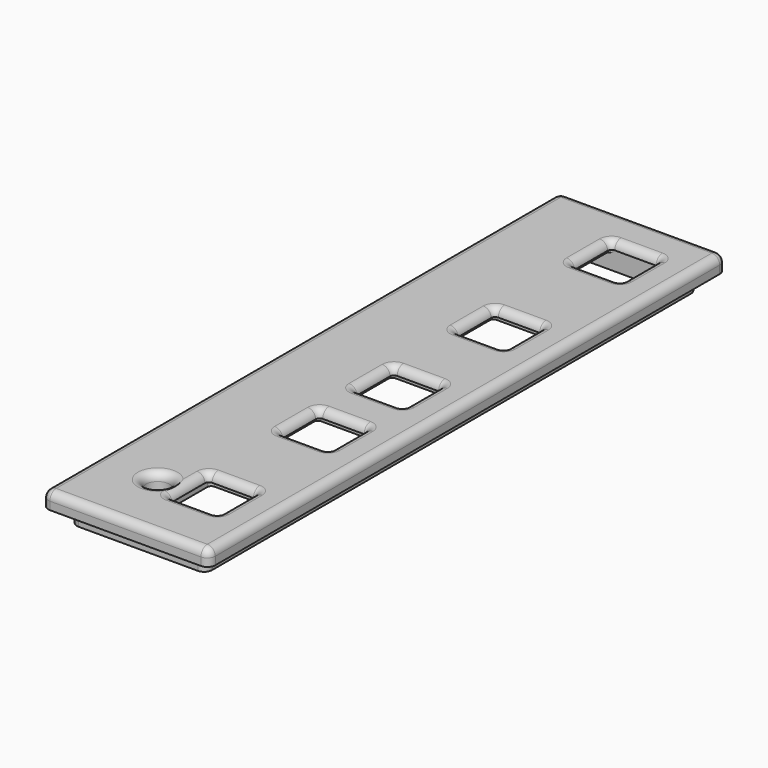
from build123d import *

# Parameters (mm, degrees)
F0_W          = 21
F0_H          = 81.3
F0_W_2        = 17
F0_H_2        = 77.3
F0_W_3        = 13
F0_H_3        = 73.3
F1_DEPTH      = 2
F2_DEPTH      = 2
F3_R          = 1.5
F4_DEPTH      = 25
F5_T1_DEPTH   = 79.3
F5_T3_DEPTH   = 19
F5_T5_DEPTH   = 5.2
F5_T7_DEPTH   = 5.2
F5_T9_DEPTH   = 5.2
F5_T11_DEPTH  = 5.2
F5_T13_DEPTH  = 5.2
F5_T15_DEPTH  = 5.2
F5_T17_DEPTH  = 3.5
F5_T19_DEPTH  = 4.5
F5_S23_W      = 1
F5_S23_H      = 1
F5_T24_DEPTH  = 1
F5_S29_W      = 1
F5_S29_H      = 1
F5_T30_DEPTH  = 1
F5_S35_W      = 1
F5_S35_H      = 1
F5_T36_DEPTH  = 1
F5_S41_W      = 1
F5_S41_H      = 1
F5_T42_DEPTH  = 1
F5_T48_ANGLE  = 90
F5_T50_ANGLE  = 90
F5_T52_ANGLE  = 90
F5_T54_ANGLE  = 90
F5_T56_ANGLE  = 90
F5_T58_ANGLE  = 90
F5_T60_ANGLE  = 90
F5_T62_ANGLE  = 90
F5_T64_ANGLE  = 90
F5_T66_ANGLE  = 90
F5_T68_ANGLE  = 90
F5_T70_ANGLE  = 90
F5_T72_ANGLE  = 90
F5_T74_ANGLE  = 90
F5_T76_ANGLE  = 90
F5_T78_ANGLE  = 90
F5_T80_ANGLE  = 90
F5_T82_ANGLE  = 90
F5_T84_ANGLE  = 90
F5_T86_ANGLE  = 90
F7_DEPTH      = 1
F7_DEPTH_BACK = 3


# Not quite as in the source:
# - a fillet or chamfer that OpenCascade refuses, or shapes differently, is made with other operations: its cross-section is extruded or revolved along the edge and cut away or added


with BuildPart() as f1:
    # F0 (on Top) → F1 (new body)
    with BuildSketch(Plane.XY):
        Rectangle(F0_W, F0_H)
        Rectangle(F0_W_2, F0_H_2, mode=Mode.SUBTRACT)
        Rectangle(F0_W_2, F0_H_2)
        Rectangle(F0_W_3, F0_H_3, mode=Mode.SUBTRACT)
        Rectangle(F0_W_3, F0_H_3)
    extrude(amount=F1_DEPTH)

    # F0 (on Top) → F2 (join)
    with BuildSketch(Plane.XY):
        Rectangle(F0_W_2, F0_H_2)
        Rectangle(F0_W_3, F0_H_3, mode=Mode.SUBTRACT)
    extrude(amount=-F2_DEPTH)

    # F3 (on face) → F4 (cut)
    with BuildSketch(Plane.XY.offset(2)):
        with BuildLine():
            ThreePointArc((6.2, 35.15), (6.0535533906, 35.5035533906), (5.7, 35.65))
            Line((5.7, 35.65), (0.5, 35.65))
            ThreePointArc((0.5, 35.65), (0.1464466094, 35.5035533906), (0, 35.15))
            Line((0, 35.15), (0, 29.95))
            ThreePointArc((0, 29.95), (0.1464466094, 29.5964466094), (0.5, 29.45))
            Line((0.5, 29.45), (5.7, 29.45))
            ThreePointArc((5.7, 29.45), (6.0535533906, 29.5964466094), (6.2, 29.95))
            Line((6.2, 29.95), (6.2, 35.15))
        make_face()
        with BuildLine():
            ThreePointArc((6.2, 16.85), (6.0535533906, 17.2035533906), (5.7, 17.35))
            Line((5.7, 17.35), (0.5, 17.35))
            ThreePointArc((0.5, 17.35), (0.1464466094, 17.2035533906), (0, 16.85))
            Line((0, 16.85), (0, 11.65))
            ThreePointArc((0, 11.65), (0.1464466094, 11.2964466094), (0.5, 11.15))
            Line((0.5, 11.15), (5.7, 11.15))
            ThreePointArc((5.7, 11.15), (6.0535533906, 11.2964466094), (6.2, 11.65))
            Line((6.2, 11.65), (6.2, 16.85))
        make_face()
        with BuildLine():
            Line((5.7, 1.45), (0.5, 1.45))
            ThreePointArc((0.5, 1.45), (0.1464466094, 1.3035533906), (0, 0.95))
            Line((0, 0.95), (0, -4.25))
            ThreePointArc((0, -4.25), (0.1464466094, -4.6035533906), (0.5, -4.75))
            Line((0.5, -4.75), (5.7, -4.75))
            ThreePointArc((5.7, -4.75), (6.0535533906, -4.6035533906), (6.2, -4.25))
            Line((6.2, -4.25), (6.2, 0.95))
            ThreePointArc((6.2, 0.95), (6.0535533906, 1.3035533906), (5.7, 1.45))
        make_face()
        with BuildLine():
            ThreePointArc((6.2, -10.75), (6.0535533906, -10.3964466094), (5.7, -10.25))
            Line((5.7, -10.25), (0.5, -10.25))
            ThreePointArc((0.5, -10.25), (0.1464466094, -10.3964466094), (0, -10.75))
            Line((0, -10.75), (0, -15.95))
            ThreePointArc((0, -15.95), (0.1464466094, -16.3035533906), (0.5, -16.45))
            Line((0.5, -16.45), (5.7, -16.45))
            ThreePointArc((5.7, -16.45), (6.0535533906, -16.3035533906), (6.2, -15.95))
            Line((6.2, -15.95), (6.2, -10.75))
        make_face()
        with BuildLine():
            ThreePointArc((6.2, -28.15), (6.0535533906, -27.7964466094), (5.7, -27.65))
            Line((5.7, -27.65), (0.5, -27.65))
            ThreePointArc((0.5, -27.65), (0.1464466094, -27.7964466094), (0, -28.15))
            Line((0, -28.15), (0, -33.35))
            ThreePointArc((0, -33.35), (0.1464466094, -33.7035533906), (0.5, -33.85))
            Line((0.5, -33.85), (5.7, -33.85))
            ThreePointArc((5.7, -33.85), (6.0535533906, -33.7035533906), (6.2, -33.35))
            Line((6.2, -33.35), (6.2, -28.15))
        make_face()
        with Locations((-2.9, -31.95)):
            Circle(F3_R)
    extrude(amount=-F4_DEPTH, mode=Mode.SUBTRACT)

    # F5: fillet of radius 1 on 53 edges, made by hand

    # F5_s2 → F5_t1 (cut)
    with BuildSketch(Plane.XZ.offset(-39.65)):
        with BuildLine():
            ThreePointArc((10.5, 1), (10.2071067812, 1.7071067812), (9.5, 2))
            Line((9.5, 2), (10.5, 2))
            Line((10.5, 2), (10.5, 1))
        make_face()
        with BuildLine():
            ThreePointArc((-9.5, 2), (-10.2071067812, 1.7071067812), (-10.5, 1))
            Line((-10.5, 1), (-10.5, 2))
            Line((-10.5, 2), (-9.5, 2))
        make_face()
    extrude(amount=F5_T1_DEPTH, mode=Mode.SUBTRACT)

    # F5_s4 → F5_t3 (cut)
    with BuildSketch(Plane.YZ.offset(-9.5)):
        with BuildLine():
            ThreePointArc((-40.65, 1), (-40.3571067812, 1.7071067812), (-39.65, 2))
            Line((-39.65, 2), (-40.65, 2))
            Line((-40.65, 2), (-40.65, 1))
        make_face()
        with BuildLine():
            ThreePointArc((40.65, 1), (40.3571067812, 1.7071067812), (39.65, 2))
            Line((39.65, 2), (40.65, 2))
            Line((40.65, 2), (40.65, 1))
        make_face()
    extrude(amount=F5_T3_DEPTH, mode=Mode.SUBTRACT)

    # F5_s6 → F5_t5 (cut)
    with BuildSketch(Plane.XZ.offset(28.15)):
        with BuildLine():
            ThreePointArc((7.2, 2), (6.4928932188, 1.7071067812), (6.2, 1))
            Line((6.2, 1), (6.2, 2))
            Line((6.2, 2), (7.2, 2))
        make_face()
        with BuildLine():
            ThreePointArc((-1, 2), (-0.2928932188, 1.7071067812), (0, 1))
            Line((0, 1), (0, 2))
            Line((0, 2), (-1, 2))
        make_face()
    extrude(amount=F5_T5_DEPTH, mode=Mode.SUBTRACT)

    # F5_s8 → F5_t7 (cut)
    with BuildSketch(Plane.YZ.offset(0.5)):
        with BuildLine():
            ThreePointArc((-26.65, 2), (-27.3571067812, 1.7071067812), (-27.65, 1))
            Line((-27.65, 1), (-27.65, 2))
            Line((-27.65, 2), (-26.65, 2))
        make_face()
        with BuildLine():
            ThreePointArc((-34.85, 2), (-34.1428932188, 1.7071067812), (-33.85, 1))
            Line((-33.85, 1), (-33.85, 2))
            Line((-33.85, 2), (-34.85, 2))
        make_face()
        with BuildLine():
            ThreePointArc((-9.25, 2), (-9.9571067812, 1.7071067812), (-10.25, 1))
            Line((-10.25, 1), (-10.25, 2))
            Line((-10.25, 2), (-9.25, 2))
        make_face()
        with BuildLine():
            ThreePointArc((-17.45, 2), (-16.7428932188, 1.7071067812), (-16.45, 1))
            Line((-16.45, 1), (-16.45, 2))
            Line((-16.45, 2), (-17.45, 2))
        make_face()
        with BuildLine():
            ThreePointArc((2.45, 2), (1.7428932188, 1.7071067812), (1.45, 1))
            Line((1.45, 1), (1.45, 2))
            Line((1.45, 2), (2.45, 2))
        make_face()
        with BuildLine():
            ThreePointArc((-5.75, 2), (-5.0428932188, 1.7071067812), (-4.75, 1))
            Line((-4.75, 1), (-4.75, 2))
            Line((-4.75, 2), (-5.75, 2))
        make_face()
        with BuildLine():
            ThreePointArc((18.35, 2), (17.6428932188, 1.7071067812), (17.35, 1))
            Line((17.35, 1), (17.35, 2))
            Line((17.35, 2), (18.35, 2))
        make_face()
        with BuildLine():
            ThreePointArc((10.15, 2), (10.8571067812, 1.7071067812), (11.15, 1))
            Line((11.15, 1), (11.15, 2))
            Line((11.15, 2), (10.15, 2))
        make_face()
        with BuildLine():
            ThreePointArc((36.65, 2), (35.9428932188, 1.7071067812), (35.65, 1))
            Line((35.65, 1), (35.65, 2))
            Line((35.65, 2), (36.65, 2))
        make_face()
        with BuildLine():
            ThreePointArc((28.45, 2), (29.1571067812, 1.7071067812), (29.45, 1))
            Line((29.45, 1), (29.45, 2))
            Line((29.45, 2), (28.45, 2))
        make_face()
    extrude(amount=F5_T7_DEPTH, mode=Mode.SUBTRACT)

    # F5_s10 → F5_t9 (cut)
    with BuildSketch(Plane.XZ.offset(10.75)):
        with BuildLine():
            ThreePointArc((7.2, 2), (6.4928932188, 1.7071067812), (6.2, 1))
            Line((6.2, 1), (6.2, 2))
            Line((6.2, 2), (7.2, 2))
        make_face()
        with BuildLine():
            ThreePointArc((-1, 2), (-0.2928932188, 1.7071067812), (0, 1))
            Line((0, 1), (0, 2))
            Line((0, 2), (-1, 2))
        make_face()
    extrude(amount=F5_T9_DEPTH, mode=Mode.SUBTRACT)

    # F5_s12 → F5_t11 (cut)
    with BuildSketch(Plane.XZ.offset(-0.95)):
        with BuildLine():
            ThreePointArc((-1, 2), (-0.2928932188, 1.7071067812), (0, 1))
            Line((0, 1), (0, 2))
            Line((0, 2), (-1, 2))
        make_face()
        with BuildLine():
            ThreePointArc((7.2, 2), (6.4928932188, 1.7071067812), (6.2, 1))
            Line((6.2, 1), (6.2, 2))
            Line((6.2, 2), (7.2, 2))
        make_face()
    extrude(amount=F5_T11_DEPTH, mode=Mode.SUBTRACT)

    # F5_s14 → F5_t13 (cut)
    with BuildSketch(Plane.XZ.offset(-16.85)):
        with BuildLine():
            ThreePointArc((7.2, 2), (6.4928932188, 1.7071067812), (6.2, 1))
            Line((6.2, 1), (6.2, 2))
            Line((6.2, 2), (7.2, 2))
        make_face()
        with BuildLine():
            ThreePointArc((-1, 2), (-0.2928932188, 1.7071067812), (0, 1))
            Line((0, 1), (0, 2))
            Line((0, 2), (-1, 2))
        make_face()
    extrude(amount=F5_T13_DEPTH, mode=Mode.SUBTRACT)

    # F5_s16 → F5_t15 (cut)
    with BuildSketch(Plane.XZ.offset(-35.15)):
        with BuildLine():
            ThreePointArc((7.2, 2), (6.4928932188, 1.7071067812), (6.2, 1))
            Line((6.2, 1), (6.2, 2))
            Line((6.2, 2), (7.2, 2))
        make_face()
        with BuildLine():
            ThreePointArc((-1, 2), (-0.2928932188, 1.7071067812), (0, 1))
            Line((0, 1), (0, 2))
            Line((0, 2), (-1, 2))
        make_face()
    extrude(amount=F5_T15_DEPTH, mode=Mode.SUBTRACT)

    # F5_s18 → F5_t17 (cut)
    with BuildSketch(Plane.XY.offset(-2.5)):
        with BuildLine():
            ThreePointArc((10.5, -39.65), (10.2071067812, -40.3571067812), (9.5, -40.65))
            Line((9.5, -40.65), (10.5, -40.65))
            Line((10.5, -40.65), (10.5, -39.65))
        make_face()
        with BuildLine():
            ThreePointArc((-9.5, -40.65), (-10.2071067812, -40.3571067812), (-10.5, -39.65))
            Line((-10.5, -39.65), (-10.5, -40.65))
            Line((-10.5, -40.65), (-9.5, -40.65))
        make_face()
        with BuildLine():
            ThreePointArc((-9.5, 40.65), (-10.2071067812, 40.3571067812), (-10.5, 39.65))
            Line((-10.5, 39.65), (-10.5, 40.65))
            Line((-10.5, 40.65), (-9.5, 40.65))
        make_face()
        with BuildLine():
            ThreePointArc((10.5, 39.65), (10.2071067812, 40.3571067812), (9.5, 40.65))
            Line((9.5, 40.65), (10.5, 40.65))
            Line((10.5, 40.65), (10.5, 39.65))
        make_face()
    extrude(amount=F5_T17_DEPTH, mode=Mode.SUBTRACT)

    # F5_s20 → F5_t19 (cut)
    with BuildSketch(Plane.XY.offset(-4.5)):
        with BuildLine():
            ThreePointArc((8.5, 37.65), (8.2071067812, 38.3571067812), (7.5, 38.65))
            Line((7.5, 38.65), (8.5, 38.65))
            Line((8.5, 38.65), (8.5, 37.65))
        make_face()
        with BuildLine():
            ThreePointArc((-7.5, 38.65), (-8.2071067812, 38.3571067812), (-8.5, 37.65))
            Line((-8.5, 37.65), (-8.5, 38.65))
            Line((-8.5, 38.65), (-7.5, 38.65))
        make_face()
        with BuildLine():
            ThreePointArc((8.5, -37.65), (8.2071067812, -38.3571067812), (7.5, -38.65))
            Line((7.5, -38.65), (8.5, -38.65))
            Line((8.5, -38.65), (8.5, -37.65))
        make_face()
        with BuildLine():
            ThreePointArc((-8.5, -37.65), (-8.2071067812, -38.3571067812), (-7.5, -38.65))
            Line((-7.5, -38.65), (-8.5, -38.65))
            Line((-8.5, -38.65), (-8.5, -37.65))
        make_face()
    extrude(amount=F5_T19_DEPTH, mode=Mode.SUBTRACT)


with BuildPart() as f5_tool22:
    # F5_s23 → F5_t24 (new body)
    with BuildSketch(Plane.YZ.offset(9.5)):
        with Locations((-40.15, 1.5)):
            Rectangle(F5_S23_W, F5_S23_H)
    extrude(amount=F5_T24_DEPTH)

    # F5_s25 → F5_t26 (revolve, cut)
    with BuildSketch(Plane(origin=(9.5, -39.65, 1), x_dir=(0, 0.7071067812, -0.7071067812), z_dir=(0, -0.7071067812, -0.7071067812))):
        with BuildLine():
            ThreePointArc((0, -1), (1, 0), (0, 1))
            Line((0, 1), (0, -1))
        make_face()
    revolve(axis=Axis((9.5, -39.65, 1), (1, 0, 0)), mode=Mode.SUBTRACT)


with BuildPart() as f1_1:
    add(f1.part)

    # F5_t21: cut F5_tool22
    add(f5_tool22.part, mode=Mode.SUBTRACT)


with BuildPart() as f5_tool28:
    # F5_s29 → F5_t30 (new body)
    with BuildSketch(Plane.YZ.offset(9.5)):
        with Locations((40.15, 1.5)):
            Rectangle(F5_S29_W, F5_S29_H)
    extrude(amount=F5_T30_DEPTH)

    # F5_s31 → F5_t32 (revolve, cut)
    with BuildSketch(Plane(origin=(9.5, 39.65, 1), x_dir=(0, -0.7071067812, -0.7071067812), z_dir=(0, -0.7071067812, 0.7071067812))):
        with BuildLine():
            ThreePointArc((0, -1), (1, 0), (0, 1))
            Line((0, 1), (0, -1))
        make_face()
    revolve(axis=Axis((9.5, 39.65, 1), (1, 0, 0)), mode=Mode.SUBTRACT)


with BuildPart() as f1_2:
    add(f1_1.part)

    # F5_t27: cut F5_tool28
    add(f5_tool28.part, mode=Mode.SUBTRACT)


with BuildPart() as f5_tool34:
    # F5_s35 → F5_t36 (new body)
    with BuildSketch(Plane.XZ.offset(39.65)):
        with Locations((-10, 1.5)):
            Rectangle(F5_S35_W, F5_S35_H)
    extrude(amount=F5_T36_DEPTH)

    # F5_s37 → F5_t38 (revolve, cut)
    with BuildSketch(Plane(origin=(-9.5, -39.65, 1), x_dir=(0.7071067812, 0, -0.7071067812), z_dir=(-0.7071067812, 0, -0.7071067812))):
        with BuildLine():
            ThreePointArc((0, -1), (1, 0), (0, 1))
            Line((0, 1), (0, -1))
        make_face()
    revolve(axis=Axis((-9.5, -39.65, 1), (0, -1, 0)), mode=Mode.SUBTRACT)


with BuildPart() as f1_3:
    add(f1_2.part)

    # F5_t33: cut F5_tool34
    add(f5_tool34.part, mode=Mode.SUBTRACT)


with BuildPart() as f5_tool40:
    # F5_s41 → F5_t42 (new body)
    with BuildSketch(Plane.XZ.offset(-39.65)):
        with Locations((-10, 1.5)):
            Rectangle(F5_S41_W, F5_S41_H)
    extrude(amount=-F5_T42_DEPTH)

    # F5_s43 → F5_t44 (revolve, cut)
    with BuildSketch(Plane(origin=(-9.5, 39.65, 1), x_dir=(0.7071067812, 0, -0.7071067812), z_dir=(0.7071067812, 0, 0.7071067812))):
        with BuildLine():
            ThreePointArc((0, -1), (1, 0), (0, 1))
            Line((0, 1), (0, -1))
        make_face()
    revolve(axis=Axis((-9.5, 39.65, 1), (0, 1, 0)), mode=Mode.SUBTRACT)


with BuildPart() as f1_4:
    add(f1_3.part)

    # F5_t39: cut F5_tool40
    add(f5_tool40.part, mode=Mode.SUBTRACT)

    # F5_s45 → F5_t46 (revolve, cut)
    with BuildSketch(Plane.XZ.offset(31.95)):
        with BuildLine():
            ThreePointArc((-0.4, 2), (-1.1071067812, 1.7071067812), (-1.4, 1))
            Line((-1.4, 1), (-1.4, 2))
            Line((-1.4, 2), (-0.4, 2))
        make_face()
    revolve(axis=Axis((-2.9, -31.95, 2), (0, 0, 1)), mode=Mode.SUBTRACT)

    # F5_s47 → F5_t48 (revolve, cut)
    with BuildSketch(Plane.XZ.offset(28.15)):
        with BuildLine():
            ThreePointArc((7.2, 2), (6.4928932188, 1.7071067812), (6.2, 1))
            Line((6.2, 1), (6.2, 2))
            Line((6.2, 2), (7.2, 2))
        make_face()
    revolve(axis=Axis((5.7, -28.15, 2), (0, 0, 1)), revolution_arc=F5_T48_ANGLE, mode=Mode.SUBTRACT)

    # F5_s49 → F5_t50 (revolve, cut)
    with BuildSketch(Plane.YZ.offset(0.5)):
        with BuildLine():
            ThreePointArc((-26.65, 2), (-27.3571067812, 1.7071067812), (-27.65, 1))
            Line((-27.65, 1), (-27.65, 2))
            Line((-27.65, 2), (-26.65, 2))
        make_face()
    revolve(axis=Axis((0.5, -28.15, 2), (0, 0, 1)), revolution_arc=F5_T50_ANGLE, mode=Mode.SUBTRACT)

    # F5_s51 → F5_t52 (revolve, cut)
    with BuildSketch(Plane.XZ.offset(33.35)):
        with BuildLine():
            ThreePointArc((-1, 2), (-0.2928932188, 1.7071067812), (0, 1))
            Line((0, 1), (0, 2))
            Line((0, 2), (-1, 2))
        make_face()
    revolve(axis=Axis((0.5, -33.35, 2), (0, 0, 1)), revolution_arc=F5_T52_ANGLE, mode=Mode.SUBTRACT)

    # F5_s53 → F5_t54 (revolve, cut)
    with BuildSketch(Plane.YZ.offset(5.7)):
        with BuildLine():
            ThreePointArc((-34.85, 2), (-34.1428932188, 1.7071067812), (-33.85, 1))
            Line((-33.85, 1), (-33.85, 2))
            Line((-33.85, 2), (-34.85, 2))
        make_face()
    revolve(axis=Axis((5.7, -33.35, 2), (0, 0, 1)), revolution_arc=F5_T54_ANGLE, mode=Mode.SUBTRACT)

    # F5_s55 → F5_t56 (revolve, cut)
    with BuildSketch(Plane.XZ.offset(10.75)):
        with BuildLine():
            ThreePointArc((7.2, 2), (6.4928932188, 1.7071067812), (6.2, 1))
            Line((6.2, 1), (6.2, 2))
            Line((6.2, 2), (7.2, 2))
        make_face()
    revolve(axis=Axis((5.7, -10.75, 2), (0, 0, 1)), revolution_arc=F5_T56_ANGLE, mode=Mode.SUBTRACT)

    # F5_s57 → F5_t58 (revolve, cut)
    with BuildSketch(Plane.YZ.offset(0.5)):
        with BuildLine():
            ThreePointArc((-9.25, 2), (-9.9571067812, 1.7071067812), (-10.25, 1))
            Line((-10.25, 1), (-10.25, 2))
            Line((-10.25, 2), (-9.25, 2))
        make_face()
    revolve(axis=Axis((0.5, -10.75, 2), (0, 0, 1)), revolution_arc=F5_T58_ANGLE, mode=Mode.SUBTRACT)

    # F5_s59 → F5_t60 (revolve, cut)
    with BuildSketch(Plane.XZ.offset(15.95)):
        with BuildLine():
            ThreePointArc((-1, 2), (-0.2928932188, 1.7071067812), (0, 1))
            Line((0, 1), (0, 2))
            Line((0, 2), (-1, 2))
        make_face()
    revolve(axis=Axis((0.5, -15.95, 2), (0, 0, 1)), revolution_arc=F5_T60_ANGLE, mode=Mode.SUBTRACT)

    # F5_s61 → F5_t62 (revolve, cut)
    with BuildSketch(Plane.YZ.offset(5.7)):
        with BuildLine():
            ThreePointArc((-17.45, 2), (-16.7428932188, 1.7071067812), (-16.45, 1))
            Line((-16.45, 1), (-16.45, 2))
            Line((-16.45, 2), (-17.45, 2))
        make_face()
    revolve(axis=Axis((5.7, -15.95, 2), (0, 0, 1)), revolution_arc=F5_T62_ANGLE, mode=Mode.SUBTRACT)

    # F5_s63 → F5_t64 (revolve, cut)
    with BuildSketch(Plane.YZ.offset(0.5)):
        with BuildLine():
            ThreePointArc((2.45, 2), (1.7428932188, 1.7071067812), (1.45, 1))
            Line((1.45, 1), (1.45, 2))
            Line((1.45, 2), (2.45, 2))
        make_face()
    revolve(axis=Axis((0.5, 0.95, 2), (0, 0, 1)), revolution_arc=F5_T64_ANGLE, mode=Mode.SUBTRACT)

    # F5_s65 → F5_t66 (revolve, cut)
    with BuildSketch(Plane.XZ.offset(4.25)):
        with BuildLine():
            ThreePointArc((-1, 2), (-0.2928932188, 1.7071067812), (0, 1))
            Line((0, 1), (0, 2))
            Line((0, 2), (-1, 2))
        make_face()
    revolve(axis=Axis((0.5, -4.25, 2), (0, 0, 1)), revolution_arc=F5_T66_ANGLE, mode=Mode.SUBTRACT)

    # F5_s67 → F5_t68 (revolve, cut)
    with BuildSketch(Plane.YZ.offset(5.7)):
        with BuildLine():
            ThreePointArc((-5.75, 2), (-5.0428932188, 1.7071067812), (-4.75, 1))
            Line((-4.75, 1), (-4.75, 2))
            Line((-4.75, 2), (-5.75, 2))
        make_face()
    revolve(axis=Axis((5.7, -4.25, 2), (0, 0, 1)), revolution_arc=F5_T68_ANGLE, mode=Mode.SUBTRACT)

    # F5_s69 → F5_t70 (revolve, cut)
    with BuildSketch(Plane.XZ.offset(-0.95)):
        with BuildLine():
            ThreePointArc((7.2, 2), (6.4928932188, 1.7071067812), (6.2, 1))
            Line((6.2, 1), (6.2, 2))
            Line((6.2, 2), (7.2, 2))
        make_face()
    revolve(axis=Axis((5.7, 0.95, 2), (0, 0, 1)), revolution_arc=F5_T70_ANGLE, mode=Mode.SUBTRACT)

    # F5_s71 → F5_t72 (revolve, cut)
    with BuildSketch(Plane.XZ.offset(-16.85)):
        with BuildLine():
            ThreePointArc((7.2, 2), (6.4928932188, 1.7071067812), (6.2, 1))
            Line((6.2, 1), (6.2, 2))
            Line((6.2, 2), (7.2, 2))
        make_face()
    revolve(axis=Axis((5.7, 16.85, 2), (0, 0, 1)), revolution_arc=F5_T72_ANGLE, mode=Mode.SUBTRACT)

    # F5_s73 → F5_t74 (revolve, cut)
    with BuildSketch(Plane.YZ.offset(0.5)):
        with BuildLine():
            ThreePointArc((18.35, 2), (17.6428932188, 1.7071067812), (17.35, 1))
            Line((17.35, 1), (17.35, 2))
            Line((17.35, 2), (18.35, 2))
        make_face()
    revolve(axis=Axis((0.5, 16.85, 2), (0, 0, 1)), revolution_arc=F5_T74_ANGLE, mode=Mode.SUBTRACT)

    # F5_s75 → F5_t76 (revolve, cut)
    with BuildSketch(Plane.XZ.offset(-11.65)):
        with BuildLine():
            ThreePointArc((-1, 2), (-0.2928932188, 1.7071067812), (0, 1))
            Line((0, 1), (0, 2))
            Line((0, 2), (-1, 2))
        make_face()
    revolve(axis=Axis((0.5, 11.65, 2), (0, 0, 1)), revolution_arc=F5_T76_ANGLE, mode=Mode.SUBTRACT)

    # F5_s77 → F5_t78 (revolve, cut)
    with BuildSketch(Plane.YZ.offset(5.7)):
        with BuildLine():
            ThreePointArc((10.15, 2), (10.8571067812, 1.7071067812), (11.15, 1))
            Line((11.15, 1), (11.15, 2))
            Line((11.15, 2), (10.15, 2))
        make_face()
    revolve(axis=Axis((5.7, 11.65, 2), (0, 0, 1)), revolution_arc=F5_T78_ANGLE, mode=Mode.SUBTRACT)

    # F5_s79 → F5_t80 (revolve, cut)
    with BuildSketch(Plane.XZ.offset(-35.15)):
        with BuildLine():
            ThreePointArc((7.2, 2), (6.4928932188, 1.7071067812), (6.2, 1))
            Line((6.2, 1), (6.2, 2))
            Line((6.2, 2), (7.2, 2))
        make_face()
    revolve(axis=Axis((5.7, 35.15, 2), (0, 0, 1)), revolution_arc=F5_T80_ANGLE, mode=Mode.SUBTRACT)

    # F5_s81 → F5_t82 (revolve, cut)
    with BuildSketch(Plane.YZ.offset(0.5)):
        with BuildLine():
            ThreePointArc((36.65, 2), (35.9428932188, 1.7071067812), (35.65, 1))
            Line((35.65, 1), (35.65, 2))
            Line((35.65, 2), (36.65, 2))
        make_face()
    revolve(axis=Axis((0.5, 35.15, 2), (0, 0, 1)), revolution_arc=F5_T82_ANGLE, mode=Mode.SUBTRACT)

    # F5_s83 → F5_t84 (revolve, cut)
    with BuildSketch(Plane.XZ.offset(-29.95)):
        with BuildLine():
            ThreePointArc((-1, 2), (-0.2928932188, 1.7071067812), (0, 1))
            Line((0, 1), (0, 2))
            Line((0, 2), (-1, 2))
        make_face()
    revolve(axis=Axis((0.5, 29.95, 2), (0, 0, 1)), revolution_arc=F5_T84_ANGLE, mode=Mode.SUBTRACT)

    # F5_s85 → F5_t86 (revolve, cut)
    with BuildSketch(Plane.YZ.offset(5.7)):
        with BuildLine():
            ThreePointArc((28.45, 2), (29.1571067812, 1.7071067812), (29.45, 1))
            Line((29.45, 1), (29.45, 2))
            Line((29.45, 2), (28.45, 2))
        make_face()
    revolve(axis=Axis((5.7, 29.95, 2), (0, 0, 1)), revolution_arc=F5_T86_ANGLE, mode=Mode.SUBTRACT)

    # F6 (on face) → F7 (cut, two sides)
    with BuildSketch(Plane.XY) as f7_sk:
        with BuildLine():
            Line((6.5, -26.65), (0, -26.65))
            ThreePointArc((0, -26.65), (-0.3535533906, -26.7964466094), (-0.5, -27.15))
            Line((-0.5, -27.15), (-0.5, -34.35))
            ThreePointArc((-0.5, -34.35), (-0.3535533906, -34.7035533906), (0, -34.85))
            Line((0, -34.85), (6.5, -34.85))
            Line((6.5, -34.85), (6.5, -26.65))
        make_face()
        with BuildLine():
            Line((7.2, -26.65), (6.5, -26.65))
            Line((6.5, -26.65), (6.5, -34.85))
            Line((6.5, -34.85), (7.2, -34.85))
            ThreePointArc((7.2, -34.85), (7.5535533906, -34.7035533906), (7.7, -34.35))
            Line((7.7, -34.35), (7.7, -27.15))
            ThreePointArc((7.7, -27.15), (7.5535533906, -26.7964466094), (7.2, -26.65))
        make_face()
        with BuildLine():
            Line((-0.5, -17.45), (6.5, -17.45))
            Line((6.5, -17.45), (6.5, -9.25))
            Line((6.5, -9.25), (-0.5, -9.25))
            ThreePointArc((-0.5, -9.25), (-0.8535533906, -9.3964466094), (-1, -9.75))
            Line((-1, -9.75), (-1, -16.95))
            ThreePointArc((-1, -16.95), (-0.8535533906, -17.3035533906), (-0.5, -17.45))
        make_face()
        with BuildLine():
            Line((6.5, -9.25), (6.5, -17.45))
            Line((6.5, -17.45), (6.7, -17.45))
            ThreePointArc((6.7, -17.45), (7.0535533906, -17.3035533906), (7.2, -16.95))
            Line((7.2, -16.95), (7.2, -9.75))
            ThreePointArc((7.2, -9.75), (7.0535533906, -9.3964466094), (6.7, -9.25))
            Line((6.7, -9.25), (6.5, -9.25))
        make_face()
        with BuildLine():
            Line((-0.5, -5.75), (6.5, -5.75))
            Line((6.5, -5.75), (6.5, 2.45))
            Line((6.5, 2.45), (-0.5, 2.45))
            ThreePointArc((-0.5, 2.45), (-0.8535533906, 2.3035533906), (-1, 1.95))
            Line((-1, 1.95), (-1, -5.25))
            ThreePointArc((-1, -5.25), (-0.8535533906, -5.6035533906), (-0.5, -5.75))
        make_face()
        with BuildLine():
            Line((6.5, 2.45), (6.5, -5.75))
            Line((6.5, -5.75), (6.7, -5.75))
            ThreePointArc((6.7, -5.75), (7.0535533906, -5.6035533906), (7.2, -5.25))
            Line((7.2, -5.25), (7.2, 1.95))
            ThreePointArc((7.2, 1.95), (7.0535533906, 2.3035533906), (6.7, 2.45))
            Line((6.7, 2.45), (6.5, 2.45))
        make_face()
        with BuildLine():
            Line((-0.5, 10.15), (6.5, 10.15))
            Line((6.5, 10.15), (6.5, 18.35))
            Line((6.5, 18.35), (-0.5, 18.35))
            ThreePointArc((-0.5, 18.35), (-0.8535533906, 18.2035533906), (-1, 17.85))
            Line((-1, 17.85), (-1, 10.65))
            ThreePointArc((-1, 10.65), (-0.8535533906, 10.2964466094), (-0.5, 10.15))
        make_face()
        with BuildLine():
            Line((6.5, 18.35), (6.5, 10.15))
            Line((6.5, 10.15), (6.7, 10.15))
            ThreePointArc((6.7, 10.15), (7.0535533906, 10.2964466094), (7.2, 10.65))
            Line((7.2, 10.65), (7.2, 17.85))
            ThreePointArc((7.2, 17.85), (7.0535533906, 18.2035533906), (6.7, 18.35))
            Line((6.7, 18.35), (6.5, 18.35))
        make_face()
        with BuildLine():
            Line((6.5, 36.65), (-0.5, 36.65))
            ThreePointArc((-0.5, 36.65), (-0.8535533906, 36.5035533906), (-1, 36.15))
            Line((-1, 36.15), (-1, 28.95))
            ThreePointArc((-1, 28.95), (-0.8535533906, 28.5964466094), (-0.5, 28.45))
            Line((-0.5, 28.45), (6.5, 28.45))
            Line((6.5, 28.45), (6.5, 36.65))
        make_face()
        with BuildLine():
            Line((6.7, 36.65), (6.5, 36.65))
            Line((6.5, 36.65), (6.5, 28.45))
            Line((6.5, 28.45), (6.7, 28.45))
            ThreePointArc((6.7, 28.45), (7.0535533906, 28.5964466094), (7.2, 28.95))
            Line((7.2, 28.95), (7.2, 36.15))
            ThreePointArc((7.2, 36.15), (7.0535533906, 36.5035533906), (6.7, 36.65))
        make_face()
    extrude(amount=F7_DEPTH, mode=Mode.SUBTRACT)
    extrude(f7_sk.sketch, amount=-F7_DEPTH_BACK, mode=Mode.SUBTRACT)


solid = f1_4.part
